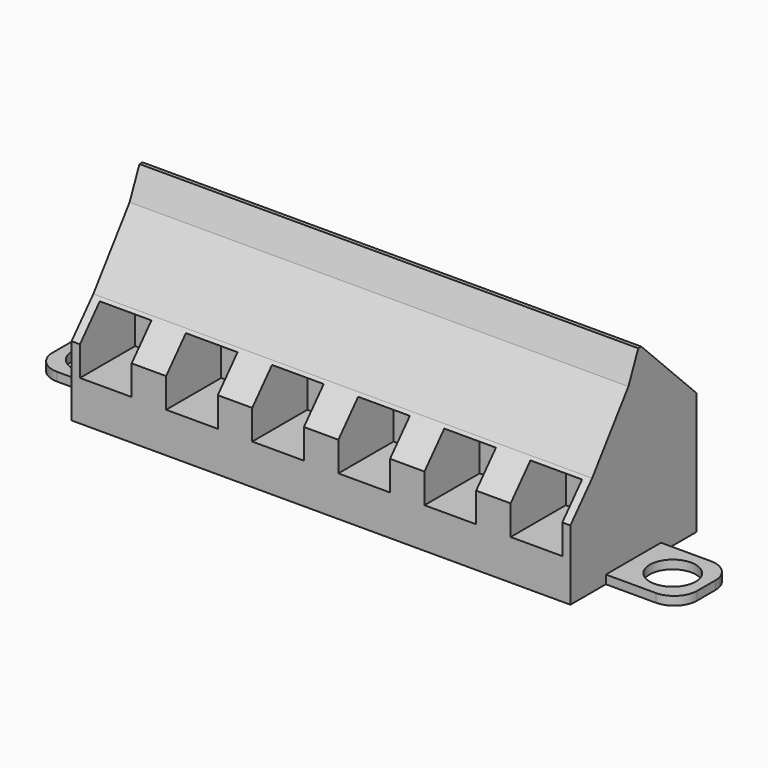
from build123d import *

# Parameters (mm, degrees)
F0_W      = 43.434
F0_H      = 13.716
F1_DEPTH  = 16.657
F3_DEPTH  = 43.435
F4_W      = 4.5
F4_H      = 5
F5_DEPTH  = 6
F6_R      = 2.25
F7_DEPTH  = 2
F8_W      = 6
F8_H      = 0.75
F9_DEPTH  = 6.35
F10_W     = 6
F10_H     = 0.75
F11_DEPTH = 6.35
F12_R     = 2
F13_R     = 2
F14_DEPTH = 0.751
F15_R     = 2
F16_DEPTH = 0.751


# Not quite as in the source:
# - a feature names something its author has since deleted; it is built from what else it names


with BuildPart() as f1:
    # F0 (on Top) → F1 (new body)
    with BuildSketch(Plane.XY):
        Rectangle(F0_W, F0_H)
    extrude(amount=F1_DEPTH)

    # F2 (on face) → F3 (cut, through all)
    with BuildSketch(Plane(origin=(-21.717, 0, 0), x_dir=(0, -1, 0), z_dir=(-1, 0, 0))):
        Polygon((-6.858, 10.657), (-0.858, 16.657), (-6.858, 16.657), align=None)
        Polygon((6.858, 16.657), (-0.5295271985, 16.657), (0.5445904681, 14.1634047031), (4.491972737, 8.7391110137), (6.858, 6.0806702822), align=None)
    extrude(amount=-F3_DEPTH, mode=Mode.SUBTRACT)

    # F4 (on face) → F5 (cut)
    with BuildSketch(Plane.XZ.offset(6.858)):
        with Locations((-18.737, 6)):
            Rectangle(F4_W, F4_H)
        with Locations((-11.237, 6)):
            Rectangle(F4_W, F4_H)
        with Locations((-3.737, 6)):
            Rectangle(F4_W, F4_H)
        with Locations((3.763, 6)):
            Rectangle(F4_W, F4_H)
        with Locations((11.263, 6)):
            Rectangle(F4_W, F4_H)
        with Locations((18.763, 6)):
            Rectangle(F4_W, F4_H)
        with Locations((26.263, 6)):
            Rectangle(F4_W, F4_H)
        with Locations((33.763, 6)):
            Rectangle(F4_W, F4_H)
        with Locations((41.263, 6)):
            Rectangle(F4_W, F4_H)
        with Locations((48.763, 6)):
            Rectangle(F4_W, F4_H)
        with Locations((56.263, 6)):
            Rectangle(F4_W, F4_H)
        with Locations((63.763, 6)):
            Rectangle(F4_W, F4_H)
    extrude(amount=-F5_DEPTH, mode=Mode.SUBTRACT)

    # F6 (on face) → F7 (cut)
    with BuildSketch(Plane(origin=(0, 8.7575, 8.7575), x_dir=(1, 0, 0), z_dir=(0, 0.7071067812, 0.7071067812))):
        with Locations((-18.737, -6.9289393488)):
            Circle(F6_R)
        with Locations((-11.237, -6.9289393488)):
            Circle(F6_R)
        with Locations((-3.737, -6.9289393488)):
            Circle(F6_R)
        with Locations((3.763, -6.9289393488)):
            Circle(F6_R)
        with Locations((11.263, -6.9289393488)):
            Circle(F6_R)
        with Locations((18.763, -6.9289393488)):
            Circle(F6_R)
        with Locations((26.263, -6.9289393488)):
            Circle(F6_R)
        with Locations((33.763, -6.9289393488)):
            Circle(F6_R)
        with Locations((41.263, -6.9289393488)):
            Circle(F6_R)
        with Locations((48.763, -6.9289393488)):
            Circle(F6_R)
        with Locations((56.263, -6.9289393488)):
            Circle(F6_R)
        with Locations((63.763, -6.9289393488)):
            Circle(F6_R)
    extrude(amount=-F7_DEPTH, mode=Mode.SUBTRACT)

    # F8 (on face) → F9 (join)
    with BuildSketch(Plane(origin=(-21.717, 0, 0), x_dir=(0, -1, 0), z_dir=(-1, 0, 0))):
        with Locations((0, 0.375)):
            Rectangle(F8_W, F8_H)
    extrude(amount=F9_DEPTH)

    # F10 (on face) → F11 (join)
    with BuildSketch(Plane.YZ.offset(21.717)):
        with Locations((0, 0.375)):
            Rectangle(F10_W, F10_H)
    extrude(amount=F11_DEPTH)

    # F12
    f12_edges = [f1.edges().sort_by_distance(p)[0] for p in [
        (-28.067, 3, 0.375),
        (-28.067, -3, 0.375),
        (28.067, -3, 0.375),
        (28.067, 3, 0.375),
    ]]
    fillet(f12_edges, radius=F12_R)

    # F13 (on face) → F14 (cut, through all)
    with BuildSketch(Plane.XY.offset(0.75)):
        with Locations((-25.1435, 0)):
            Circle(F13_R)
    extrude(amount=-F14_DEPTH, mode=Mode.SUBTRACT)

    # F15 (on face) → F16 (cut, through all)
    with BuildSketch(Plane.XY.offset(0.75)):
        with Locations((25.1435, 0)):
            Circle(F15_R)
    extrude(amount=-F16_DEPTH, mode=Mode.SUBTRACT)


solid = f1.part
